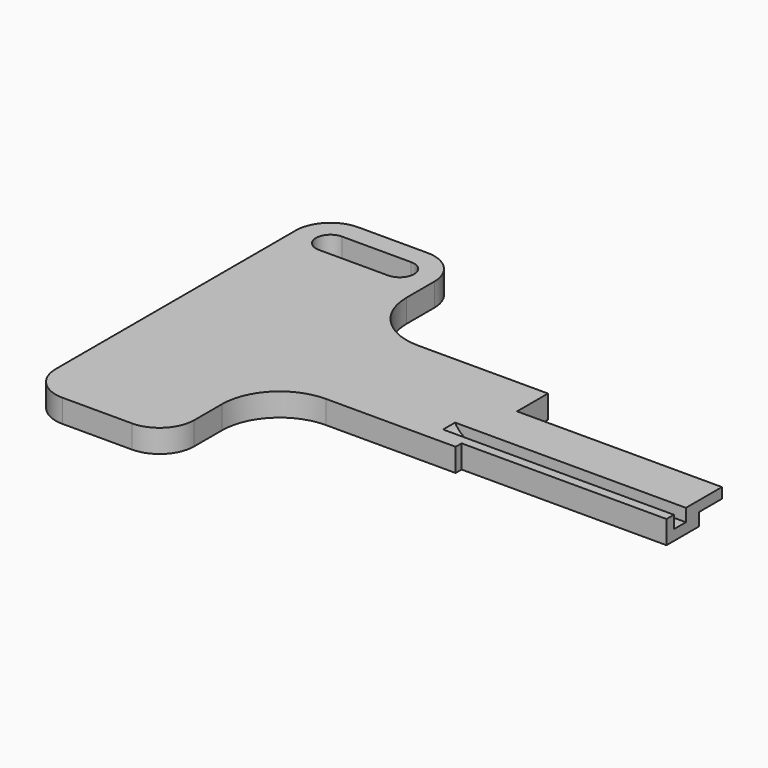
from build123d import *

# Parameters (mm, degrees)
F1_DEPTH    = 2
F2_W        = 1.3
F2_H        = 1.1
F2_W_2      = 2.5
F3_DEPTH    = 20
F4_T1_DEPTH = 1.3
F5_T4_DEPTH = 6.9651427749


# Not quite as in the source:
# - a fillet or chamfer that OpenCascade refuses, or shapes differently, is made with other operations: its cross-section is extruded or revolved along the edge and cut away or added


with BuildPart() as f1:
    # F0 (on Top) → F1 (new body)
    with BuildSketch(Plane.XY):
        with BuildLine():
            ThreePointArc((0, 3), (0.8786796564, 0.8786796564), (3, 0))
            Line((3, 0), (9, 0))
            ThreePointArc((9, 0), (11.1213203436, 0.8786796564), (12, 3))
            Line((12, 3), (12, 6))
            ThreePointArc((12, 6), (13.4644660941, 9.5355339059), (17, 11))
            Line((17, 11), (28.25, 11))
            Line((28.25, 11), (28.25, 11.65))
            Line((28.25, 11.65), (46, 11.65))
            Line((46, 11.65), (46, 17.65))
            Line((46, 17.65), (28.25, 17.65))
            Line((28.25, 17.65), (28.25, 21))
            Line((28.25, 21), (17, 21))
            ThreePointArc((17, 21), (13.4644660941, 22.4644660941), (12, 26))
            Line((12, 26), (12, 29))
            ThreePointArc((12, 29), (11.1213203436, 31.1213203436), (9, 32))
            Line((9, 32), (3, 32))
            ThreePointArc((3, 32), (0.8786796564, 31.1213203436), (0, 29))
            Line((0, 29), (0, 3))
        make_face()
        with BuildLine():
            ThreePointArc((3, 27.75), (1.75, 29), (3, 30.25))
            Line((3, 30.25), (9, 30.25))
            ThreePointArc((9, 30.25), (10.25, 29), (9, 27.75))
            Line((9, 27.75), (3, 27.75))
        make_face(mode=Mode.SUBTRACT)
    extrude(amount=F1_DEPTH)

    # F2 (on face) → F3 (cut)
    with BuildSketch(Plane.YZ.offset(46)):
        with Locations((13.1, 1.45)):
            Rectangle(F2_W, F2_H)
        with Locations((16.4, 0.55)):
            Rectangle(F2_W_2, F2_H)
    extrude(amount=-F3_DEPTH, mode=Mode.SUBTRACT)

    # F4: fillet of radius 2 on 1 edges, made by hand

    # F4_s2 → F4_t1 (join)
    with BuildSketch(Plane.XZ.offset(-13.75)):
        with BuildLine():
            ThreePointArc((26, 2), (26.7372482618, 1.1970613634), (27.7860571099, 0.9))
            Line((27.7860571099, 0.9), (26, 0.9))
            Line((26, 0.9), (26, 2))
        make_face()
    extrude(amount=F4_T1_DEPTH)

    # F5: fillet of radius 2 on 1 edges, made by hand


with BuildPart() as f5_tool2:
    # F5_s3 → F5_t4 (new body)
    with BuildSketch(Plane.XZ.offset(-17.65)):
        with BuildLine():
            ThreePointArc((26, 0), (26.7372482618, 0.8029386366), (27.7860571099, 1.1))
            Line((27.7860571099, 1.1), (26, 1.1))
            Line((26, 1.1), (26, 0))
        make_face()
    extrude(amount=F5_T4_DEPTH)

    split(bisect_by=Plane.XZ.offset(-13.75), keep=Keep.BOTTOM)


with BuildPart() as f1_1:
    add(f1.part)

    # F5_t1: union F5_tool2
    add(f5_tool2.part)


solid = f1_1.part
